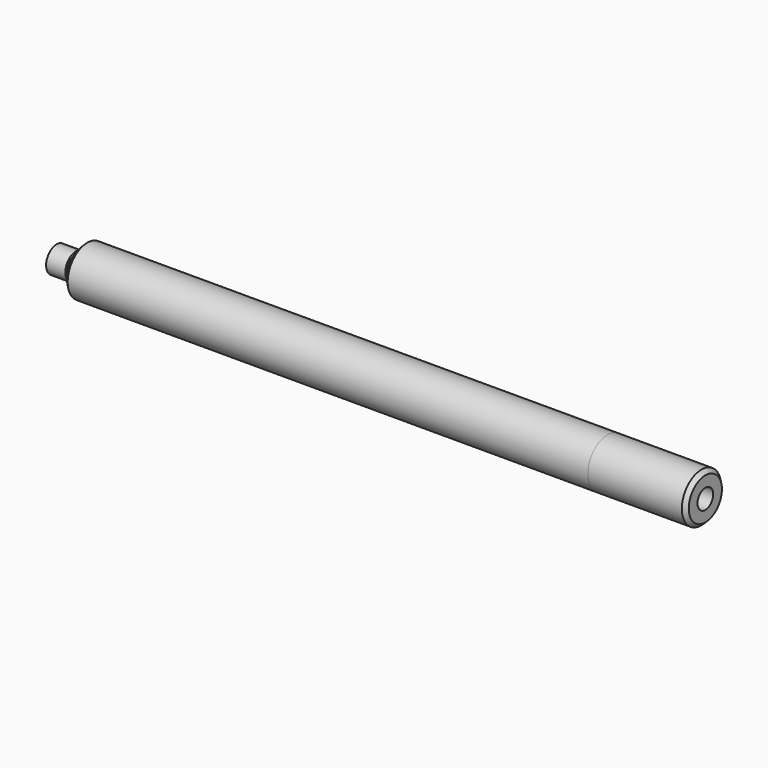
from build123d import *

# Parameters (mm, degrees)
F0_R      = 6.4
F1_DEPTH  = 25.5
F3_D      = 5.1
F4_R      = 6.4
F4_R_2    = 2.55
F5_DEPTH  = 136.5
F6_SIZE2  = 1
F6_SIZE   = 1
F7_R      = 2.7297634072
F8_DEPTH  = 7
F9_R      = 3.4275534108
F10_DEPTH = 5


with BuildPart() as f1:
    # F0 (on Right) → F1 (new body)
    with BuildSketch(Plane.YZ):
        Circle(F0_R)
    extrude(amount=-F1_DEPTH)

    # F3 (through all)
    with Locations(Plane.YZ):
        with Locations((0, 0)):
            Hole(F3_D / 2)

    # F4 (on face) → F5 (join)
    with BuildSketch(Plane(origin=(-25.5, 0, 0), x_dir=(0, -1, 0), z_dir=(-1, 0, 0))):
        Circle(F4_R)
        Circle(F4_R_2, mode=Mode.SUBTRACT)
        Circle(F4_R_2)
    extrude(amount=F5_DEPTH)

    # F6
    f6_edges = [f1.edges().sort_by_distance(p)[0] for p in [
        (0, -6.4, 0),
        (-12.75, 6.4, 0),
        (-25.5, 0, -6.4),
        (-25.5, 0, 6.4),
        (-93.75, -6.4, 0),
        (-162, 6.4, 0),
    ]]
    chamfer(f6_edges, length=F6_SIZE, length2=F6_SIZE2)

    # F7 (on face) → F8 (join)
    with BuildSketch(Plane(origin=(-162, 0, 0), x_dir=(0, -1, 0), z_dir=(-1, 0, 0))):
        Circle(F7_R)
    extrude(amount=F8_DEPTH)

    # F9 (on face) → F10 (join)
    with BuildSketch(Plane(origin=(-169, 0, 0), x_dir=(0, -1, 0), z_dir=(-1, 0, 0))):
        Circle(F9_R)
    extrude(amount=-F10_DEPTH)


solid = f1.part
